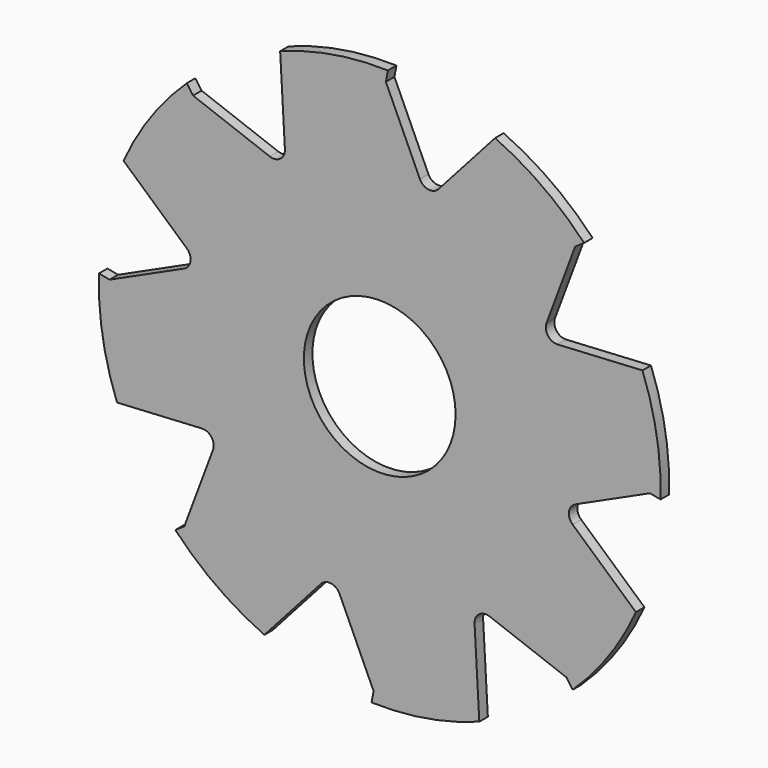
from build123d import *

# Parameters (mm, degrees)
F0_R            = 50
F0_R_2          = 13.5
F1_DEPTH        = 1.9
F3_DEPTH        = 25
F5_DEPTH        = 25
F5_COPIES_COUNT = 8


# Not quite as in the source:
# - a pattern or mirror of a feature is missing from the dataset's text; its kind, count and spacing are read off the source's solid


with BuildPart() as f1:
    # F0 (on Front) → F1 (new body)
    with BuildSketch(Plane.XZ):
        Circle(F0_R)
        Circle(F0_R_2, mode=Mode.SUBTRACT)
    extrude(amount=F1_DEPTH)

    # F2 (on Front) → F3 (cut)
    with BuildSketch(Plane.XZ):
        with BuildLine():
            Line((12.4794095755, 60.955286026), (0, 50.1961745322))
            Line((0, 50.1961745322), (2.7271706326, 35.8238514012))
            ThreePointArc((2.7271706326, 35.8238514012), (3.9364062163, 34.3449689954), (5.8350966322, 34.555488762))
            Line((5.8350966322, 34.555488762), (21.0234094411, 45.1330654323))
            Line((21.0234094411, 45.1330654323), (12.4794095755, 60.955286026))
        make_face()
    extrude(amount=-F3_DEPTH, mode=Mode.SUBTRACT)

    # F4 (on Front) → F5 (cut)
    with BuildSketch(Plane.XZ):
        with BuildLine():
            Line((10.4537707273, 34.3168952742), (22.7111335844, 48.0314604938))
            Line((22.7111335844, 48.0314604938), (18.2506803442, 59.0550513337))
            Line((18.2506803442, 59.0550513337), (1.7007282507, 51.2778109993))
            Line((1.7007282507, 51.2778109993), (1.0944613384, 48.079281378))
            Line((1.0944613384, 48.079281378), (7.1429279991, 34.8196319836))
            ThreePointArc((7.1429279991, 34.8196319836), (8.6623060706, 33.6723315481), (10.4537707273, 34.3168952742))
        make_face()
    f5 = extrude(amount=F5_DEPTH, mode=Mode.SUBTRACT)

    # F5_copies: F5 ×8 about axis
    f5_copies_axis = Axis((0, 0, 0), (0, 1, 0))
    for i in range(1, F5_COPIES_COUNT):
        add(f5.rotate(f5_copies_axis, i * 360 / F5_COPIES_COUNT), mode=Mode.SUBTRACT)


solid = f1.part
